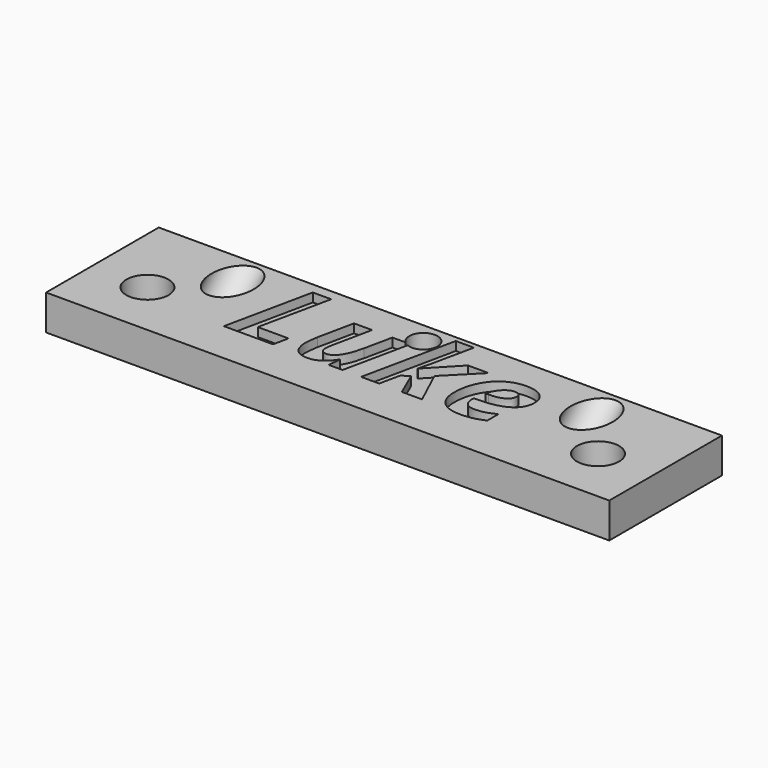
from build123d import *

# Parameters (mm, degrees)
F0_W         = 101.6
F0_H         = 25.4
F1_DEPTH     = 6.35
F2_R         = 3.81
F3_DEPTH     = 25.4
F7_R         = 3.81
F8_DEPTH     = 62.8627928475
F9_TEXT_SIZE = 22.212201954
F10_DEPTH    = 1.5875
F11_R        = 2.54
F12_DEPTH    = 25.4


# Not quite as in the source:
# - Text() gives the source's letters only with a copy of the font that has no kerning and outlines rounded to 1/6400 em; it was checked with that copy


with BuildPart() as f1:
    # F0 (on Top) → F1 (new body)
    with BuildSketch(Plane.XY):
        Rectangle(F0_W, F0_H)
    extrude(amount=F1_DEPTH)

    # F2 (on face) → F3 (cut)
    with BuildSketch(Plane.XY.offset(6.35)):
        with Locations((-40.64, -2.54)):
            Circle(F2_R)
        with Locations((40.64, -2.54)):
            Circle(F2_R)
    extrude(amount=-F3_DEPTH, mode=Mode.SUBTRACT)

    # F7 (on 3pt) → F8 (cut, through all)
    with BuildSketch(Plane(origin=(0, 38.1, 38.1), x_dir=(1, 0, 0), z_dir=(0, -0.7071067812, -0.7071067812))):
        with Locations((-32.385, 0)):
            Circle(F7_R)
        with Locations((32.385, 0)):
            Circle(F7_R)
    extrude(amount=F8_DEPTH, mode=Mode.SUBTRACT)

    # F9 (on face) → F10 (cut)
    with BuildSketch(Plane.XY.offset(6.35)):
        with Locations((-25.4, -5.08)):
            Text('Luke', F9_TEXT_SIZE, font='Open Sans', font_style=FontStyle.BOLDITALIC, text_align=(TextAlign.LEFT, TextAlign.BOTTOM))
    extrude(amount=-F10_DEPTH, mode=Mode.SUBTRACT)

    # F11 (on face) → F12 (cut)
    with BuildSketch(Plane(origin=(0, 0, 0), x_dir=(1, 0, 0), z_dir=(0, 0, -1))):
        with Locations((0, -8.89)):
            Circle(F11_R)
    extrude(amount=-F12_DEPTH, mode=Mode.SUBTRACT)


solid = f1.part
